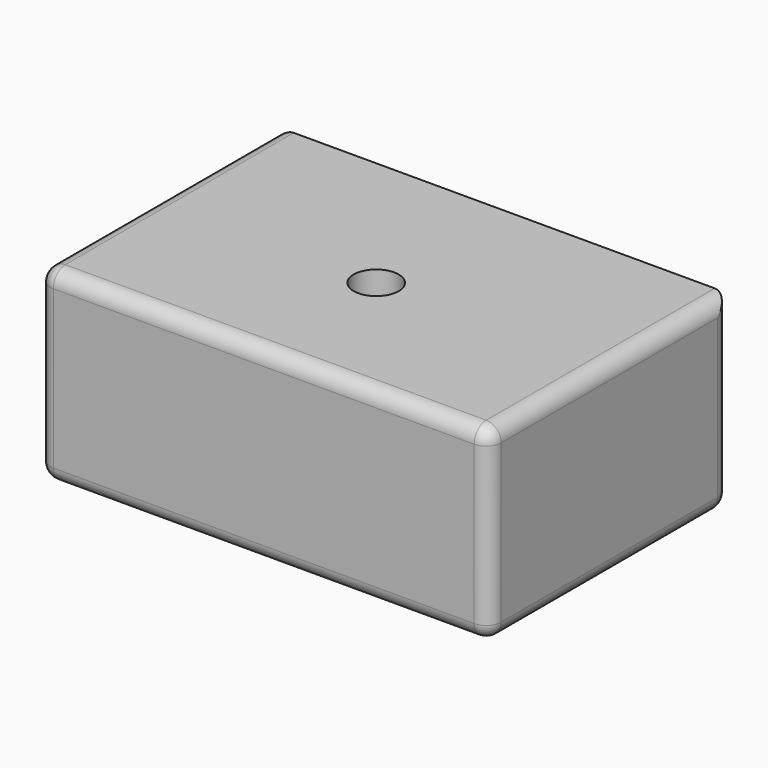
from build123d import *

# Parameters (mm, degrees)
F0_W         = 300
F0_H         = 200
F0_R         = 15
F1_DEPTH     = 25
F2_DEPTH     = 100
F3_R         = 10
F6_T1_DEPTH  = 105
F6_T3_DEPTH  = 180
F6_T5_DEPTH  = 130
F6_T7_DEPTH  = 280
F6_T9_DEPTH  = 140
F6_T11_DEPTH = 215
F6_S15_W     = 10.2
F6_S15_H     = 10.2
F6_T16_DEPTH = 10.2
F6_S21_W     = 10.2
F6_S21_H     = 10.2
F6_T22_DEPTH = 10.2
F6_S27_W     = 10.2
F6_S27_H     = 10.2
F6_T28_DEPTH = 10.2
F6_S33_W     = 10.2
F6_S33_H     = 10.2
F6_T34_DEPTH = 10.2
F6_S39_W     = 10.2
F6_S39_H     = 10.2
F6_T40_DEPTH = 10.2
F6_T44_ANGLE = 90


# Not quite as in the source:
# - a fillet or chamfer that OpenCascade refuses, or shapes differently, is made with other operations: its cross-section is extruded or revolved along the edge and cut away or added
# - a feature of the source that left no trace in its solid (it failed there, or was rolled back) is left out


with BuildPart() as f1:
    # F0 (on Top) → F1 (new body)
    with BuildSketch(Plane.XY):
        with Locations((-0.7391218096, 3.9163683355)):
            Rectangle(F0_W, F0_H)
        with Locations((-1.9179330509, -1.0798395535)):
            Circle(F0_R, mode=Mode.SUBTRACT)
    extrude(amount=F1_DEPTH)

    # F0 (on Top) → F2 (join)
    with BuildSketch(Plane.XY):
        with Locations((-0.7391218096, 3.9163683355)):
            Rectangle(F0_W, F0_H)
        with Locations((-1.9179330509, -1.0798395535)):
            Circle(F0_R, mode=Mode.SUBTRACT)
    extrude(amount=-F2_DEPTH)

    # F3
    f3_edges = [f1.edges().sort_by_distance(p)[0] for p in [
        (-150.739122, 3.916368, 25),
    ]]
    fillet(f3_edges, radius=F3_R)

    # F6: fillet of radius 10 on 11 edges, made by hand

    # F6_s2 → F6_t1 (cut)
    with BuildSketch(Plane.XY.offset(-90)):
        with BuildLine():
            ThreePointArc((-150.7391218096, -86.0836316645), (-147.8101896215, -93.1546994763), (-140.7391218096, -96.0836316645))
            Line((-140.7391218096, -96.0836316645), (-150.7391218096, -96.0836316645))
            Line((-150.7391218096, -96.0836316645), (-150.7391218096, -86.0836316645))
        make_face()
        with BuildLine():
            ThreePointArc((139.2608781904, -96.0836316645), (146.3319460023, -93.1546994763), (149.2608781904, -86.0836316645))
            Line((149.2608781904, -86.0836316645), (149.2608781904, -96.0836316645))
            Line((149.2608781904, -96.0836316645), (139.2608781904, -96.0836316645))
        make_face()
    extrude(amount=F6_T1_DEPTH, mode=Mode.SUBTRACT)

    # F6_s4 → F6_t3 (cut)
    with BuildSketch(Plane.XZ.offset(-93.9163683355)):
        with BuildLine():
            ThreePointArc((-150.7391218096, -90), (-147.8101896215, -97.0710678119), (-140.7391218096, -100))
            Line((-140.7391218096, -100), (-150.7391218096, -100))
            Line((-150.7391218096, -100), (-150.7391218096, -90))
        make_face()
        with BuildLine():
            ThreePointArc((139.2608781904, -100), (146.3319460023, -97.0710678119), (149.2608781904, -90))
            Line((149.2608781904, -90), (149.2608781904, -100))
            Line((149.2608781904, -100), (139.2608781904, -100))
        make_face()
    extrude(amount=F6_T3_DEPTH, mode=Mode.SUBTRACT)

    # F6_s6 → F6_t5 (cut)
    with BuildSketch(Plane.XY.offset(-90)):
        with BuildLine():
            ThreePointArc((-150.7391218096, 93.9163683355), (-147.8101896215, 100.9874361474), (-140.7391218096, 103.9163683355))
            Line((-140.7391218096, 103.9163683355), (-150.7391218096, 103.9163683355))
            Line((-150.7391218096, 103.9163683355), (-150.7391218096, 93.9163683355))
        make_face()
    extrude(amount=F6_T5_DEPTH, mode=Mode.SUBTRACT)

    # F6_s8 → F6_t7 (cut)
    with BuildSketch(Plane.YZ.offset(-140.7391218096)):
        with BuildLine():
            ThreePointArc((-96.0836316645, -90), (-93.1546994763, -97.0710678119), (-86.0836316645, -100))
            Line((-86.0836316645, -100), (-96.0836316645, -100))
            Line((-96.0836316645, -100), (-96.0836316645, -90))
        make_face()
        with BuildLine():
            ThreePointArc((-96.0836316645, 15), (-93.1546994763, 22.0710678119), (-86.0836316645, 25))
            Line((-86.0836316645, 25), (-96.0836316645, 25))
            Line((-96.0836316645, 25), (-96.0836316645, 15))
        make_face()
        with BuildLine():
            ThreePointArc((93.9163683355, -100), (100.9874361474, -97.0710678119), (103.9163683355, -90))
            Line((103.9163683355, -90), (103.9163683355, -100))
            Line((103.9163683355, -100), (93.9163683355, -100))
        make_face()
    extrude(amount=F6_T7_DEPTH, mode=Mode.SUBTRACT)

    # F6_s10 → F6_t9 (cut)
    with BuildSketch(Plane.XY.offset(-90)):
        with BuildLine():
            ThreePointArc((139.2608781904, 103.9163683355), (146.3319460023, 100.9874361474), (149.2608781904, 93.9163683355))
            Line((149.2608781904, 93.9163683355), (149.2608781904, 103.9163683355))
            Line((149.2608781904, 103.9163683355), (139.2608781904, 103.9163683355))
        make_face()
    extrude(amount=F6_T9_DEPTH, mode=Mode.SUBTRACT)

    # F6_s12 → F6_t11 (cut)
    with BuildSketch(Plane.XZ.offset(-128.9163683355)):
        with BuildLine():
            ThreePointArc((139.2608781904, 25), (146.3319460023, 22.0710678119), (149.2608781904, 15))
            Line((149.2608781904, 15), (149.2608781904, 25))
            Line((149.2608781904, 25), (139.2608781904, 25))
        make_face()
    extrude(amount=F6_T11_DEPTH, mode=Mode.SUBTRACT)


with BuildPart() as f6_tool14:
    # F6_s15 → F6_t16 (new body)
    with BuildSketch(Plane.YZ.offset(-140.7391218096)):
        with Locations((-91.1836316645, -95.1)):
            Rectangle(F6_S15_W, F6_S15_H)
    extrude(amount=-F6_T16_DEPTH)

    # F6_s17 → F6_t18 (revolve, cut)
    with BuildSketch(Plane(origin=(-140.7391218096, -86.0836316645, -90), x_dir=(0, 0.7071067812, 0.7071067812), z_dir=(0, -0.7071067812, 0.7071067812))):
        with BuildLine():
            ThreePointArc((0, -10), (10, 0), (0, 10))
            Line((0, 10), (0, -10))
        make_face()
    revolve(axis=Axis((-140.7391218096, -86.0836316645, -90), (-1, 0, 0)), mode=Mode.SUBTRACT)


with BuildPart() as f1_1:
    add(f1.part)

    # F6_t13: cut F6_tool14
    add(f6_tool14.part, mode=Mode.SUBTRACT)


with BuildPart() as f6_tool20:
    # F6_s21 → F6_t22 (new body)
    with BuildSketch(Plane.YZ.offset(-140.7391218096)):
        with Locations((99.0163683355, -95.1)):
            Rectangle(F6_S21_W, F6_S21_H)
    extrude(amount=-F6_T22_DEPTH)

    # F6_s23 → F6_t24 (revolve, cut)
    with BuildSketch(Plane(origin=(-140.7391218096, 93.9163683355, -90), x_dir=(0, -0.7071067812, 0.7071067812), z_dir=(0, -0.7071067812, -0.7071067812))):
        with BuildLine():
            ThreePointArc((0, -10), (10, 0), (0, 10))
            Line((0, 10), (0, -10))
        make_face()
    revolve(axis=Axis((-140.7391218096, 93.9163683355, -90), (-1, 0, 0)), mode=Mode.SUBTRACT)


with BuildPart() as f1_2:
    add(f1_1.part)

    # F6_t19: cut F6_tool20
    add(f6_tool20.part, mode=Mode.SUBTRACT)


with BuildPart() as f6_tool26:
    # F6_s27 → F6_t28 (new body)
    with BuildSketch(Plane.XZ.offset(86.0836316645)):
        with Locations((144.3608781904, -95.1)):
            Rectangle(F6_S27_W, F6_S27_H)
    extrude(amount=F6_T28_DEPTH)

    # F6_s29 → F6_t30 (revolve, cut)
    with BuildSketch(Plane(origin=(139.2608781904, -86.0836316645, -90), x_dir=(-0.7071067812, 0, 0.7071067812), z_dir=(0.7071067812, 0, 0.7071067812))):
        with BuildLine():
            ThreePointArc((0, -10), (10, 0), (0, 10))
            Line((0, 10), (0, -10))
        make_face()
    revolve(axis=Axis((139.2608781904, -86.0836316645, -90), (0, -1, 0)), mode=Mode.SUBTRACT)


with BuildPart() as f1_3:
    add(f1_2.part)

    # F6_t25: cut F6_tool26
    add(f6_tool26.part, mode=Mode.SUBTRACT)


with BuildPart() as f6_tool32:
    # F6_s33 → F6_t34 (new body)
    with BuildSketch(Plane.XZ.offset(86.0836316645)):
        with Locations((144.3608781904, 20.1)):
            Rectangle(F6_S33_W, F6_S33_H)
    extrude(amount=F6_T34_DEPTH)

    # F6_s35 → F6_t36 (revolve, cut)
    with BuildSketch(Plane(origin=(139.2608781904, -86.0836316645, 15), x_dir=(-0.7071067812, 0, -0.7071067812), z_dir=(-0.7071067812, 0, 0.7071067812))):
        with BuildLine():
            ThreePointArc((0, -10), (10, 0), (0, 10))
            Line((0, 10), (0, -10))
        make_face()
    revolve(axis=Axis((139.2608781904, -86.0836316645, 15), (0, -1, 0)), mode=Mode.SUBTRACT)


with BuildPart() as f1_4:
    add(f1_3.part)

    # F6_t31: cut F6_tool32
    add(f6_tool32.part, mode=Mode.SUBTRACT)


with BuildPart() as f6_tool38:
    # F6_s39 → F6_t40 (new body)
    with BuildSketch(Plane.XY.offset(-90)):
        with Locations((144.3608781904, 99.0163683355)):
            Rectangle(F6_S39_W, F6_S39_H)
    extrude(amount=-F6_T40_DEPTH)

    # F6_s41 → F6_t42 (revolve, cut)
    with BuildSketch(Plane(origin=(139.2608781904, 93.9163683355, -90), x_dir=(-0.7071067812, -0.7071067812, 0), z_dir=(0.7071067812, -0.7071067812, 0))):
        with BuildLine():
            ThreePointArc((0, -10), (10, 0), (0, 10))
            Line((0, 10), (0, -10))
        make_face()
    revolve(axis=Axis((139.2608781904, 93.9163683355, -90), (0, 0, -1)), mode=Mode.SUBTRACT)


with BuildPart() as f1_5:
    add(f1_4.part)

    # F6_t37: cut F6_tool38
    add(f6_tool38.part, mode=Mode.SUBTRACT)

    # F6_s43 → F6_t44 (revolve, cut)
    with BuildSketch(Plane.XY.offset(15)):
        with BuildLine():
            ThreePointArc((-140.7391218096, -96.0836316645), (-147.8101896215, -93.1546994763), (-150.7391218096, -86.0836316645))
            Line((-150.7391218096, -86.0836316645), (-150.7391218096, -96.0836316645))
            Line((-150.7391218096, -96.0836316645), (-140.7391218096, -96.0836316645))
        make_face()
    revolve(axis=Axis((-140.7391218096, -96.0836316645, 15), (0, 1, 0)), revolution_arc=F6_T44_ANGLE, mode=Mode.SUBTRACT)


solid = f1_5.part
